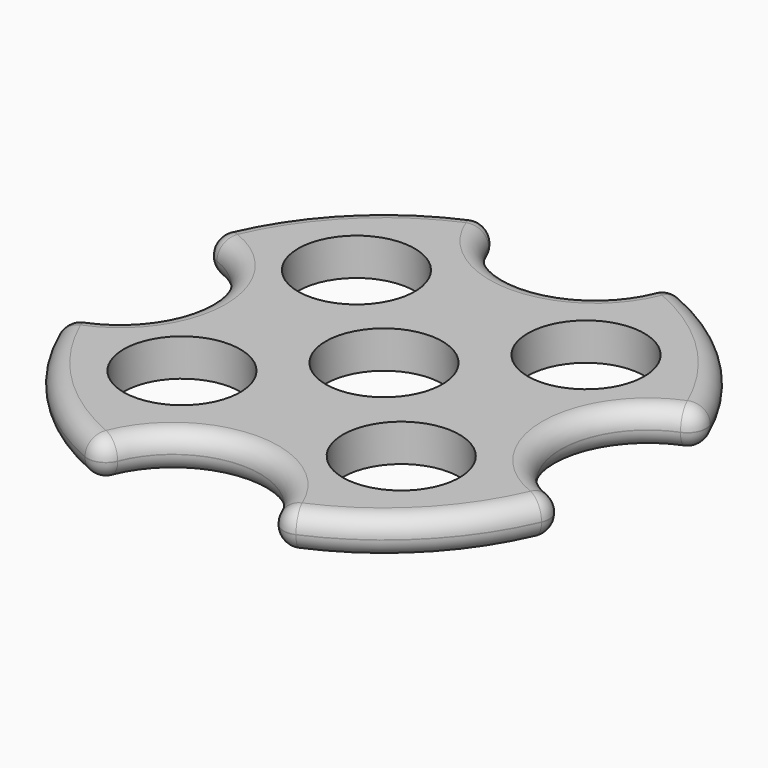
from build123d import *

# Parameters (mm, degrees)
F0_R     = 50
F1_DEPTH = 7.075
F2_D     = 22.075
F2_DEPTH = 35.375
F2_TIP   = 6.6319990825
F3_D     = 33
F3_DEPTH = 35.375
F3_TIP   = 9.914200214
F4_R     = 3.5


with BuildPart() as f1:
    # F0 (on Top) → F1 (new body)
    with BuildSketch(Plane.XY):
        Circle(F0_R)
    extrude(amount=F1_DEPTH)

    # F2
    with Locations(Plane(origin=(0, 0, 0), x_dir=(1, 0, 0), z_dir=(0, 0, -1))):
        with Locations((0, 0), (-21.75, -20.6624659709), (21.75, -20.6624659709), (20.6624659709, 21.75), (-21.75, 20.6624659709)):
            Hole(F2_D / 2, depth=F2_DEPTH)
            with Locations((0, 0, -(F2_DEPTH + F2_TIP / 2))):  # 118° drill point
                Cone(0, F2_D / 2, F2_TIP, mode=Mode.SUBTRACT)

    # F3
    with Locations(Plane(origin=(0, 0, 0), x_dir=(1, 0, 0), z_dir=(0, 0, -1))):
        with Locations((0, 50), (-50, 0), (0, -50), (50, 0)):
            Hole(F3_D / 2, depth=F3_DEPTH)
            with Locations((0, 0, -(F3_DEPTH + F3_TIP / 2))):  # 118° drill point
                Cone(0, F3_D / 2, F3_TIP, mode=Mode.SUBTRACT)

    # F4
    f4_edges = [f1.edges().sort_by_distance(p)[0] for p in [
        (35.355339, 35.355339, 0),
        (16.273844, 47.2775, 3.5375),
        (35.355339, 35.355339, 7.075),
        (47.2775, 16.273844, 3.5375),
        (33.5, 0, 7.075),
        (47.2775, -16.273844, 3.5375),
        (33.5, 0, 0),
        (35.355339, -35.355339, 7.075),
        (16.273844, -47.2775, 3.5375),
        (35.355339, -35.355339, 0),
        (0, -33.5, 7.075),
        (-16.273844, -47.2775, 3.5375),
        (0, -33.5, 0),
        (-35.355339, -35.355339, 7.075),
        (-47.2775, -16.273844, 3.5375),
        (-35.355339, -35.355339, 0),
        (-33.5, 0, 0),
        (-47.2775, 16.273844, 3.5375),
        (-33.5, 0, 7.075),
        (-35.355339, 35.355339, 0),
        (-35.355339, 35.355339, 7.075),
        (-16.273844, 47.2775, 3.5375),
        (0, 33.5, 7.075),
        (0, 33.5, 0),
    ]]
    fillet(f4_edges, radius=F4_R)


solid = f1.part
